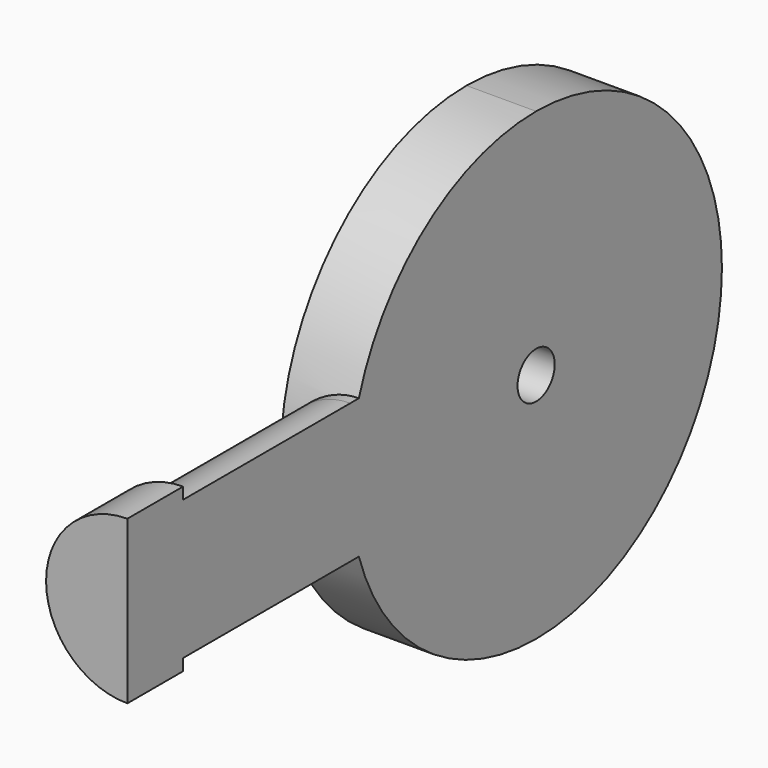
from build123d import *

# Parameters (mm, degrees)
F0_W         = 20
F0_H         = 20
F1_DEPTH     = 3
F3_DEPTH     = 9
F4_R         = 9.99999
F5_T3_DEPTH  = 53
F5_S4_R      = 3
F5_T5_DEPTH  = 29
F5_T8_DEPTH  = 53
F5_S9_R      = 3
F5_T10_DEPTH = 29
F6_R         = 1
F7_DEPTH     = 25
F9_DEPTH     = 3


# Not quite as in the source:
# - a fillet or chamfer that OpenCascade refuses, or shapes differently, is made with other operations: its cross-section is extruded or revolved along the edge and cut away or added
# - a fillet or chamfer is up to 0.001 mm smaller than in the source, because OpenCascade refuses the exact size


with BuildPart() as f1:
    # F0 (on Right) → F1 (new body)
    with BuildSketch(Plane.YZ):
        with Locations((28.7687871605, 25.2807487535)):
            Rectangle(F0_W, F0_H)
    extrude(amount=F1_DEPTH)

    # F2 (on face) → F3 (join)
    with BuildSketch(Plane.XZ.offset(-18.7687871605)):
        with BuildLine():
            Line((3, 22.2807487535), (3, 28.2807487535))
            ThreePointArc((3, 28.2807487535), (0.8786796564, 27.4020690971), (0, 25.2807487535))
            ThreePointArc((0, 25.2807487535), (0.8786796564, 23.15942841), (3, 22.2807487535))
        make_face()
    extrude(amount=F3_DEPTH)

    # F4 (radius 10 in the source; OpenCascade refuses exactly that, so slightly less here)
    f4_edges = [f1.edges().sort_by_distance(p)[0] for p in [
        (1.5, 38.768787, 35.280749),
        (1.5, 38.768787, 15.280749),
    ]]
    fillet(f4_edges, radius=F4_R)

    # F5: fillet of radius 10 on 2 edges, made by hand


with BuildPart() as f5_tool1:
    # F5_s2 → F5_t3 (new body)
    with BuildSketch(Plane.YZ.offset(-25)):
        with BuildLine():
            ThreePointArc((18.7687871605, 25.2807487535), (21.6977193487, 32.3518165654), (28.7687871605, 35.2807487535))
            Line((28.7687871605, 35.2807487535), (18.7687871605, 35.2807487535))
            Line((18.7687871605, 35.2807487535), (18.7687871605, 25.2807487535))
        make_face()
    extrude(amount=F5_T3_DEPTH)

    # F5_s4 → F5_t5 (cut, symmetric)
    with BuildSketch(Plane.XZ.offset(-23.8)):
        with Locations((3, 25.2807487535)):
            Circle(F5_S4_R)
    extrude(amount=F5_T5_DEPTH, both=True, mode=Mode.SUBTRACT)


with BuildPart() as f5_tool6:
    # F5_s7 → F5_t8 (new body)
    with BuildSketch(Plane.YZ.offset(-25)):
        with BuildLine():
            ThreePointArc((28.7687871605, 15.2807487535), (21.6977193487, 18.2096809417), (18.7687871605, 25.2807487535))
            Line((18.7687871605, 25.2807487535), (18.7687871605, 15.2807487535))
            Line((18.7687871605, 15.2807487535), (28.7687871605, 15.2807487535))
        make_face()
    extrude(amount=F5_T8_DEPTH)

    # F5_s9 → F5_t10 (cut, symmetric)
    with BuildSketch(Plane.XZ.offset(-23.8)):
        with Locations((3, 25.2807487535)):
            Circle(F5_S9_R)
    extrude(amount=F5_T10_DEPTH, both=True, mode=Mode.SUBTRACT)


with BuildPart() as f1_1:
    add(f1.part)

    # F5_t11: cut F5_tool1, F5_tool6
    add([f5_tool1.part, f5_tool6.part], mode=Mode.SUBTRACT)

    # F6 (on face) → F7 (cut)
    with BuildSketch(Plane(origin=(0, 0, 0), x_dir=(0, -1, 0), z_dir=(-1, 0, 0))):
        with Locations((-28.7687871605, 25.2807487535)):
            Circle(F6_R)
    extrude(amount=-F7_DEPTH, mode=Mode.SUBTRACT)

    # F8 (on face) → F9 (join)
    with BuildSketch(Plane.XZ.offset(-9.7687871605)):
        with BuildLine():
            Line((3, 28.2807487535), (3, 28.7807487535))
            ThreePointArc((3, 28.7807487535), (-0.5, 25.2807487535), (3, 21.7807487535))
            Line((3, 21.7807487535), (3, 22.2807487535))
            ThreePointArc((3, 22.2807487535), (0, 25.2807487535), (3, 28.2807487535))
        make_face()
        with BuildLine():
            Line((3, 22.2807487535), (3, 28.2807487535))
            ThreePointArc((3, 28.2807487535), (0, 25.2807487535), (3, 22.2807487535))
        make_face()
    extrude(amount=F9_DEPTH)


solid = f1_1.part
